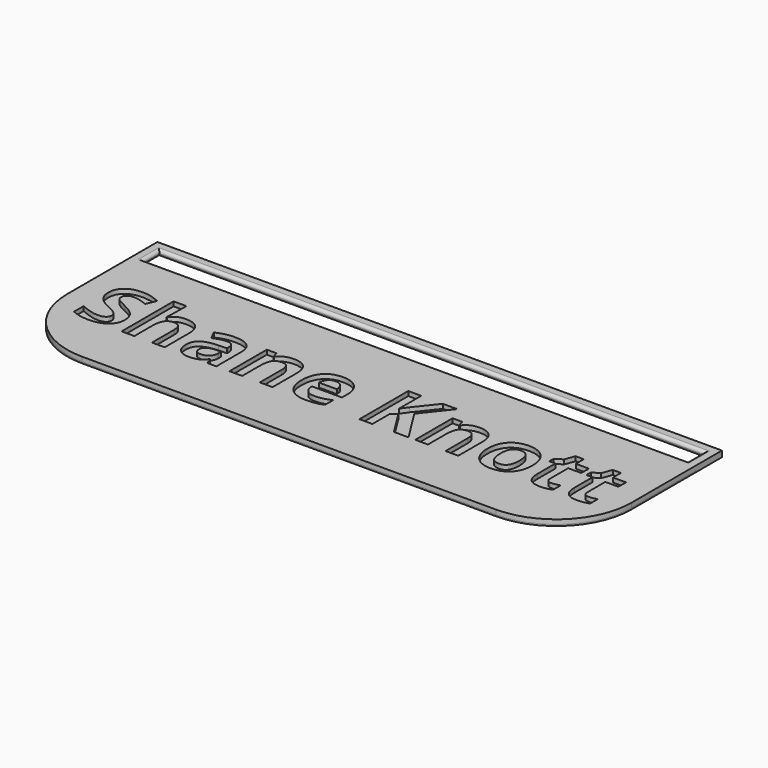
from build123d import *

# Parameters (mm, degrees)
F0_W         = 190.5
F0_H         = 63.5
F1_DEPTH     = 2
F2_W         = 183.896
F2_H         = 7.62
F3_DEPTH     = 25.4
F4_R         = 0.99999
F5_R         = 0.99999
F6_R         = 25.4
F7_TEXT_SIZE = 28.858512338
F8_DEPTH     = 2
F10_DEPTH    = 0.5


# Not quite as in the source:
# - a fillet or chamfer is up to 0.001 mm smaller than in the source, because OpenCascade refuses the exact size
# - Text() gives the source's letters only with a copy of the font that has no kerning and outlines rounded to 1/6400 em; it was checked with that copy


with BuildPart() as f1:
    # F0 (on Top) → F1 (new body)
    with BuildSketch(Plane.XY):
        with Locations((1.791532172, 31.75)):
            Rectangle(F0_W, F0_H)
    extrude(amount=F1_DEPTH)

    # F2 (on face) → F3 (cut)
    with BuildSketch(Plane.XY.offset(2)):
        with Locations((1.791532172, 56.388)):
            Rectangle(F2_W, F2_H)
    extrude(amount=-F3_DEPTH, mode=Mode.SUBTRACT)

    # F4 (radius 1 in the source; OpenCascade refuses exactly that, so slightly less here)
    f4_edges = [f1.edges().sort_by_distance(p)[0] for p in [
        (1.791532, 60.198, 2),
        (1.791532, 60.198, 0),
    ]]
    fillet(f4_edges, radius=F4_R)

    # F5 (radius 1 in the source; OpenCascade refuses exactly that, so slightly less here)
    f5_edges = [f1.edges().sort_by_distance(p)[0] for p in [
        (93.739532, 56.388, 0),
        (93.739532, 56.388, 2),
        (-90.156468, 56.388, 2),
        (-90.156468, 56.388, 0),
    ]]
    fillet(f5_edges, radius=F5_R)

    # F6
    f6_edges = [f1.edges().sort_by_distance(p)[0] for p in [
        (-93.458468, 0, 1),
        (97.041532, 0, 1),
    ]]
    fillet(f6_edges, radius=F6_R)

    # F7 (on face) → F8 (cut)
    with BuildSketch(Plane.XY.offset(2)):
        with Locations((-87.108467828, 17.78)):
            Text('Shane Knott', F7_TEXT_SIZE, font='Open Sans', font_style=FontStyle.BOLD, text_align=(TextAlign.LEFT, TextAlign.BOTTOM))
    extrude(amount=-F8_DEPTH, mode=Mode.SUBTRACT)


with BuildPart() as f10:
    # F9 (on face) → F10 (new body)
    with BuildSketch(Plane(origin=(0, 0, 0), x_dir=(1, 0, 0), z_dir=(0, 0, -1))):
        with BuildLine():
            Line((-93.458467828, -52.578), (97.041532172, -52.578))
            Line((97.041532172, -52.578), (97.041532172, -25.4))
            ThreePointArc((97.041532172, -25.4), (89.6020444142, -7.4394877579), (71.641532172, 0))
            Line((71.641532172, 0), (-68.058467828, 0))
            ThreePointArc((-68.058467828, 0), (-86.0189800701, -7.4394877579), (-93.458467828, -25.4))
            Line((-93.458467828, -25.4), (-93.458467828, -52.578))
        make_face()
    extrude(amount=-F10_DEPTH)


solid = Compound([f1.part, f10.part])
